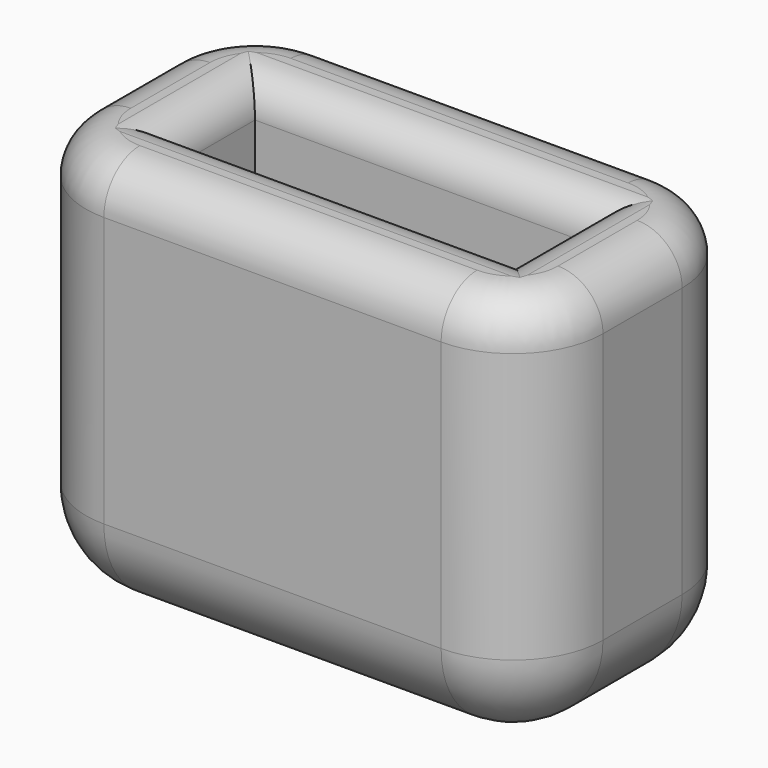
from build123d import *

# Parameters (mm, degrees)
F0_W         = 11.5
F0_H         = 6.2
F0_W_2       = 7.5
F0_H_2       = 2.2
F1_DEPTH     = 7
F2_W         = 11.5
F2_H         = 6.2
F3_DEPTH     = 2
F4_R         = 2
F5_R         = 0.8
F6_T1_DEPTH  = 2.2
F6_T3_DEPTH  = 7.5
F6_T6_ANGLE  = 90
F6_T8_ANGLE  = 90
F6_T10_ANGLE = 90
F6_T12_ANGLE = 90


# Not quite as in the source:
# - a fillet or chamfer that OpenCascade refuses, or shapes differently, is made with other operations: its cross-section is extruded or revolved along the edge and cut away or added


with BuildPart() as f1:
    # F0 (on Top) → F1 (new body)
    with BuildSketch(Plane.XY):
        Rectangle(F0_W, F0_H)
        Rectangle(F0_W_2, F0_H_2, mode=Mode.SUBTRACT)
    extrude(amount=F1_DEPTH)

    # F2 (on face) → F3 (join)
    with BuildSketch(Plane(origin=(0, 0, 0), x_dir=(1, 0, 0), z_dir=(0, 0, -1))):
        Rectangle(F2_W, F2_H)
    extrude(amount=F3_DEPTH)

    # F4
    f4_edges = [f1.edges().sort_by_distance(p)[0] for p in [
        (5.75, 0, -2),
        (0, -3.1, -2),
        (-5.75, 0, -2),
        (0, 3.1, -2),
        (5.75, -3.1, 2.5),
        (5.75, 3.1, 2.5),
        (-5.75, -3.1, 2.5),
        (-5.75, 3.1, 2.5),
    ]]
    fillet(f4_edges, radius=F4_R)

    # F5
    f5_edges = [f1.edges().sort_by_distance(p)[0] for p in [
        (0, -1.1, 7),
        (3.75, 0, 7),
        (-3.75, 0, 7),
        (0, 1.1, 7),
    ]]
    fillet(f5_edges, radius=F5_R)

    # F6: fillet of radius 1 on 8 edges, made by hand

    # F6_s2 → F6_t1 (cut)
    with BuildSketch(Plane.XZ.offset(-1.1)):
        with BuildLine():
            ThreePointArc((4.75, 7), (5.4571067812, 6.7071067812), (5.75, 6))
            Line((5.75, 6), (5.75, 7))
            Line((5.75, 7), (4.75, 7))
        make_face()
        with BuildLine():
            ThreePointArc((-4.75, 7), (-5.4571067812, 6.7071067812), (-5.75, 6))
            Line((-5.75, 6), (-5.75, 7))
            Line((-5.75, 7), (-4.75, 7))
        make_face()
    extrude(amount=F6_T1_DEPTH, mode=Mode.SUBTRACT)

    # F6_s4 → F6_t3 (cut)
    with BuildSketch(Plane.YZ.offset(-3.75)):
        with BuildLine():
            ThreePointArc((2.1, 7), (2.8071067812, 6.7071067812), (3.1, 6))
            Line((3.1, 6), (3.1, 7))
            Line((3.1, 7), (2.1, 7))
        make_face()
        with BuildLine():
            ThreePointArc((-2.1, 7), (-2.8071067812, 6.7071067812), (-3.1, 6))
            Line((-3.1, 6), (-3.1, 7))
            Line((-3.1, 7), (-2.1, 7))
        make_face()
    extrude(amount=F6_T3_DEPTH, mode=Mode.SUBTRACT)

    # F6_s5 → F6_t6 (revolve, cut)
    with BuildSketch(Plane.YZ.offset(3.75)):
        with BuildLine():
            ThreePointArc((2.1, 7), (2.8071067812, 6.7071067812), (3.1, 6))
            Line((3.1, 6), (3.1, 7))
            Line((3.1, 7), (2.1, 7))
        make_face()
    revolve(axis=Axis((3.75, 1.1, 7), (0, 0, -1)), revolution_arc=F6_T6_ANGLE, mode=Mode.SUBTRACT)

    # F6_s7 → F6_t8 (revolve, cut)
    with BuildSketch(Plane.YZ.offset(-3.75)):
        with BuildLine():
            ThreePointArc((2.1, 7), (2.8071067812, 6.7071067812), (3.1, 6))
            Line((3.1, 6), (3.1, 7))
            Line((3.1, 7), (2.1, 7))
        make_face()
    revolve(axis=Axis((-3.75, 1.1, 7), (0, 0, 1)), revolution_arc=F6_T8_ANGLE, mode=Mode.SUBTRACT)

    # F6_s9 → F6_t10 (revolve, cut)
    with BuildSketch(Plane.YZ.offset(3.75)):
        with BuildLine():
            ThreePointArc((-2.1, 7), (-2.8071067812, 6.7071067812), (-3.1, 6))
            Line((-3.1, 6), (-3.1, 7))
            Line((-3.1, 7), (-2.1, 7))
        make_face()
    revolve(axis=Axis((3.75, -1.1, 7), (0, 0, 1)), revolution_arc=F6_T10_ANGLE, mode=Mode.SUBTRACT)

    # F6_s11 → F6_t12 (revolve, cut)
    with BuildSketch(Plane.YZ.offset(-3.75)):
        with BuildLine():
            ThreePointArc((-2.1, 7), (-2.8071067812, 6.7071067812), (-3.1, 6))
            Line((-3.1, 6), (-3.1, 7))
            Line((-3.1, 7), (-2.1, 7))
        make_face()
    revolve(axis=Axis((-3.75, -1.1, 7), (0, 0, -1)), revolution_arc=F6_T12_ANGLE, mode=Mode.SUBTRACT)


solid = f1.part
